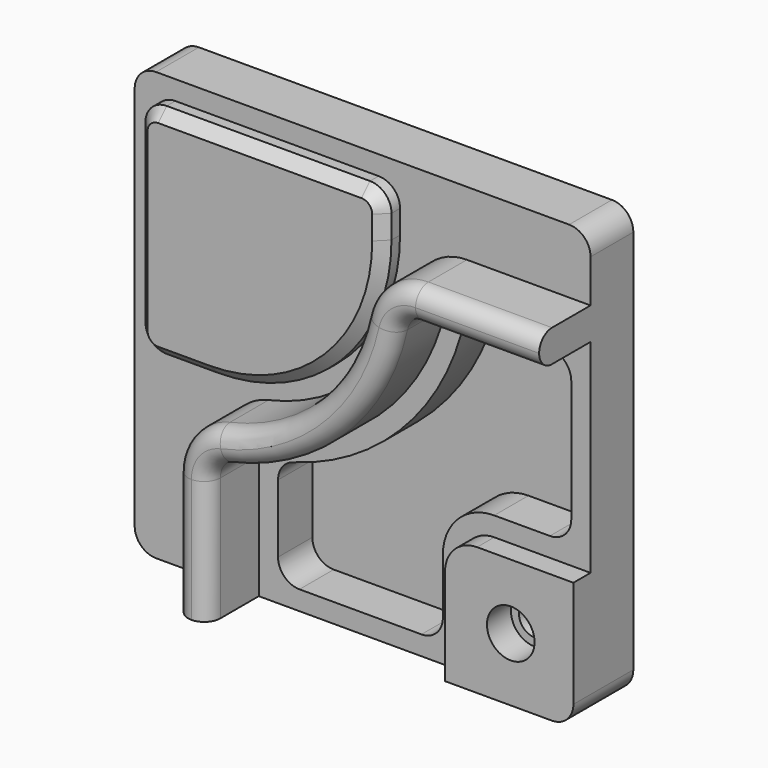
from build123d import *

# Parameters (mm, degrees)
F1_DEPTH       = 25
F2_DEPTH       = 10
F3_DEPTH       = 30
F4_DEPTH       = 20
F5_DEPTH       = 10
F7_D           = 14.75
F7_CBORE_D     = 22.25
F7_CBORE_DEPTH = 14
F8_SIZE        = 5
F9_R           = 7.49999


# Not quite as in the source:
# - a fillet or chamfer is up to 0.001 mm smaller than in the source, because OpenCascade refuses the exact size


with BuildPart() as f1:
    # F0 (on Front) → F1 (new body)
    with BuildSketch(Plane.XZ):
        with BuildLine():
            Line((96.5, 100), (-96.5, 100))
            ThreePointArc((-96.5, 100), (-103.5710678119, 97.0710678119), (-106.5, 90))
            Line((-106.5, 90), (-106.5, -90))
            ThreePointArc((-106.5, -90), (-103.5710678119, -97.0710678119), (-96.5, -100))
            Line((-96.5, -100), (-63.5, -100))
            Line((-63.5, -100), (-63.5, -42.2497216032))
            ThreePointArc((-63.5, -42.2497216032), (-58.0047374401, -26.6111405489), (-43.9347826087, -17.8476082112))
            ThreePointArc((-43.9347826087, -17.8476082112), (0.1396103068, 6.3603896932), (24.3476082112, 50.4347826087))
            ThreePointArc((24.3476082112, 50.4347826087), (33.1111405489, 64.5047374401), (48.7497216032, 70))
            Line((48.7497216032, 70), (106.5, 70))
            Line((106.5, 70), (106.5, 90))
            ThreePointArc((106.5, 90), (103.5710678119, 97.0710678119), (96.5, 100))
        make_face()
        with BuildLine():
            ThreePointArc((17.5, 70), (-6.2243507239, 12.7243507239), (-63.5, -11))
            Line((-63.5, -11), (-87.5, -11))
            ThreePointArc((-87.5, -11), (-94.5710678119, -8.0710678119), (-97.5, -1))
            Line((-97.5, -1), (-97.5, 81))
            ThreePointArc((-97.5, 81), (-94.5710678119, 88.0710678119), (-87.5, 91))
            Line((-87.5, 91), (7.5, 91))
            ThreePointArc((7.5, 91), (14.5710678119, 88.0710678119), (17.5, 81))
            Line((17.5, 81), (17.5, 70))
        make_face(mode=Mode.SUBTRACT)
        with BuildLine():
            Line((106.5, 55), (106.5, 70))
            Line((106.5, 70), (48.7497216032, 70))
            ThreePointArc((48.7497216032, 70), (33.1111405489, 64.5047374401), (24.3476082112, 50.4347826087))
            ThreePointArc((24.3476082112, 50.4347826087), (0.1396103068, 6.3603896932), (-43.9347826087, -17.8476082112))
            ThreePointArc((-43.9347826087, -17.8476082112), (-58.0047374401, -26.6111405489), (-63.5, -42.2497216032))
            Line((-63.5, -42.2497216032), (-63.5, -100))
            Line((-63.5, -100), (-48.5, -100))
            Line((-48.5, -100), (-48.5, -42.2497216032))
            ThreePointArc((-48.5, -42.2497216032), (-46.3018949761, -35.9942891815), (-40.6739130435, -32.4888762464))
            ThreePointArc((-40.6739130435, -32.4888762464), (10.7462120246, -4.2462120246), (38.9888762464, 47.1739130435))
            ThreePointArc((38.9888762464, 47.1739130435), (42.4942891815, 52.8018949761), (48.7497216032, 55))
            Line((48.7497216032, 55), (106.5, 55))
        make_face()
        with BuildLine():
            Line((106.5, -40), (106.5, 55))
            Line((106.5, 55), (48.7497216032, 55))
            ThreePointArc((48.7497216032, 55), (42.4942891815, 52.8018949761), (38.9888762464, 47.1739130435))
            ThreePointArc((38.9888762464, 47.1739130435), (10.7462120246, -4.2462120246), (-40.6739130435, -32.4888762464))
            ThreePointArc((-40.6739130435, -32.4888762464), (-46.3018949761, -35.9942891815), (-48.5, -42.2497216032))
            Line((-48.5, -42.2497216032), (-48.5, -100))
            Line((-48.5, -100), (46.5, -100))
            Line((46.5, -100), (46.5, -55))
            ThreePointArc((46.5, -55), (50.8933982822, -44.3933982822), (61.5, -40))
            Line((61.5, -40), (106.5, -40))
        make_face()
        with BuildLine():
            ThreePointArc((46.130896205, 38.7419354839), (49.7234965193, 43.981834214), (55.7476414861, 46))
            Line((55.7476414861, 46), (87.5, 46))
            ThreePointArc((87.5, 46), (94.5710678119, 43.0710678119), (97.5, 36))
            Line((97.5, 36), (97.5, -21))
            ThreePointArc((97.5, -21), (94.5710678119, -28.0710678119), (87.5, -31))
            Line((87.5, -31), (61.5, -31))
            ThreePointArc((61.5, -31), (44.5294372515, -38.0294372515), (37.5, -55))
            Line((37.5, -55), (37.5, -81))
            ThreePointArc((37.5, -81), (34.5710678119, -88.0710678119), (27.5, -91))
            Line((27.5, -91), (-29.5, -91))
            ThreePointArc((-29.5, -91), (-36.5710678119, -88.0710678119), (-39.5, -81))
            Line((-39.5, -81), (-39.5, -49.2476414861))
            ThreePointArc((-39.5, -49.2476414861), (-37.481834214, -43.2234965193), (-32.2419354839, -39.630896205))
            ThreePointArc((-32.2419354839, -39.630896205), (17.1101730553, -10.6101730553), (46.130896205, 38.7419354839))
        make_face(mode=Mode.SUBTRACT)
        with BuildLine():
            Line((106.5, -90), (106.5, -40))
            Line((106.5, -40), (61.5, -40))
            ThreePointArc((61.5, -40), (50.8933982822, -44.3933982822), (46.5, -55))
            Line((46.5, -55), (46.5, -100))
            Line((46.5, -100), (96.5, -100))
            ThreePointArc((96.5, -100), (103.5710678119, -97.0710678119), (106.5, -90))
        make_face()
        with BuildLine():
            Line((-87.5, -11), (-63.5, -11))
            ThreePointArc((-63.5, -11), (-6.2243507239, 12.7243507239), (17.5, 70))
            Line((17.5, 70), (17.5, 81))
            ThreePointArc((17.5, 81), (14.5710678119, 88.0710678119), (7.5, 91))
            Line((7.5, 91), (-87.5, 91))
            ThreePointArc((-87.5, 91), (-94.5710678119, 88.0710678119), (-97.5, 81))
            Line((-97.5, 81), (-97.5, -1))
            ThreePointArc((-97.5, -1), (-94.5710678119, -8.0710678119), (-87.5, -11))
        make_face()
        with BuildLine():
            Line((87.5, 46), (55.7476414861, 46))
            ThreePointArc((55.7476414861, 46), (49.7234965193, 43.981834214), (46.130896205, 38.7419354839))
            ThreePointArc((46.130896205, 38.7419354839), (17.1101730553, -10.6101730553), (-32.2419354839, -39.630896205))
            ThreePointArc((-32.2419354839, -39.630896205), (-37.481834214, -43.2234965193), (-39.5, -49.2476414861))
            Line((-39.5, -49.2476414861), (-39.5, -81))
            ThreePointArc((-39.5, -81), (-36.5710678119, -88.0710678119), (-29.5, -91))
            Line((-29.5, -91), (27.5, -91))
            ThreePointArc((27.5, -91), (34.5710678119, -88.0710678119), (37.5, -81))
            Line((37.5, -81), (37.5, -55))
            ThreePointArc((37.5, -55), (44.5294372515, -38.0294372515), (61.5, -31))
            Line((61.5, -31), (87.5, -31))
            ThreePointArc((87.5, -31), (94.5710678119, -28.0710678119), (97.5, -21))
            Line((97.5, -21), (97.5, 36))
            ThreePointArc((97.5, 36), (94.5710678119, 43.0710678119), (87.5, 46))
        make_face()
    extrude(amount=-F1_DEPTH)

    # F0 (on Front) → F2 (join)
    with BuildSketch(Plane.XZ):
        with BuildLine():
            Line((-87.5, -11), (-63.5, -11))
            ThreePointArc((-63.5, -11), (-6.2243507239, 12.7243507239), (17.5, 70))
            Line((17.5, 70), (17.5, 81))
            ThreePointArc((17.5, 81), (14.5710678119, 88.0710678119), (7.5, 91))
            Line((7.5, 91), (-87.5, 91))
            ThreePointArc((-87.5, 91), (-94.5710678119, 88.0710678119), (-97.5, 81))
            Line((-97.5, 81), (-97.5, -1))
            ThreePointArc((-97.5, -1), (-94.5710678119, -8.0710678119), (-87.5, -11))
        make_face()
    extrude(amount=F2_DEPTH)

    # F0 (on Front) → F3 (join)
    with BuildSketch(Plane.XZ):
        with BuildLine():
            Line((106.5, 55), (106.5, 70))
            Line((106.5, 70), (48.7497216032, 70))
            ThreePointArc((48.7497216032, 70), (33.1111405489, 64.5047374401), (24.3476082112, 50.4347826087))
            ThreePointArc((24.3476082112, 50.4347826087), (0.1396103068, 6.3603896932), (-43.9347826087, -17.8476082112))
            ThreePointArc((-43.9347826087, -17.8476082112), (-58.0047374401, -26.6111405489), (-63.5, -42.2497216032))
            Line((-63.5, -42.2497216032), (-63.5, -100))
            Line((-63.5, -100), (-48.5, -100))
            Line((-48.5, -100), (-48.5, -42.2497216032))
            ThreePointArc((-48.5, -42.2497216032), (-46.3018949761, -35.9942891815), (-40.6739130435, -32.4888762464))
            ThreePointArc((-40.6739130435, -32.4888762464), (10.7462120246, -4.2462120246), (38.9888762464, 47.1739130435))
            ThreePointArc((38.9888762464, 47.1739130435), (42.4942891815, 52.8018949761), (48.7497216032, 55))
            Line((48.7497216032, 55), (106.5, 55))
        make_face()
    extrude(amount=F3_DEPTH)

    # F0 (on Front) → F4 (cut)
    with BuildSketch(Plane.XZ):
        with BuildLine():
            Line((87.5, 46), (55.7476414861, 46))
            ThreePointArc((55.7476414861, 46), (49.7234965193, 43.981834214), (46.130896205, 38.7419354839))
            ThreePointArc((46.130896205, 38.7419354839), (17.1101730553, -10.6101730553), (-32.2419354839, -39.630896205))
            ThreePointArc((-32.2419354839, -39.630896205), (-37.481834214, -43.2234965193), (-39.5, -49.2476414861))
            Line((-39.5, -49.2476414861), (-39.5, -81))
            ThreePointArc((-39.5, -81), (-36.5710678119, -88.0710678119), (-29.5, -91))
            Line((-29.5, -91), (27.5, -91))
            ThreePointArc((27.5, -91), (34.5710678119, -88.0710678119), (37.5, -81))
            Line((37.5, -81), (37.5, -55))
            ThreePointArc((37.5, -55), (44.5294372515, -38.0294372515), (61.5, -31))
            Line((61.5, -31), (87.5, -31))
            ThreePointArc((87.5, -31), (94.5710678119, -28.0710678119), (97.5, -21))
            Line((97.5, -21), (97.5, 36))
            ThreePointArc((97.5, 36), (94.5710678119, 43.0710678119), (87.5, 46))
        make_face()
    extrude(amount=-F4_DEPTH, mode=Mode.SUBTRACT)

    # F0 (on Front) → F5 (join)
    with BuildSketch(Plane.XZ):
        with BuildLine():
            Line((106.5, -90), (106.5, -40))
            Line((106.5, -40), (61.5, -40))
            ThreePointArc((61.5, -40), (50.8933982822, -44.3933982822), (46.5, -55))
            Line((46.5, -55), (46.5, -100))
            Line((46.5, -100), (96.5, -100))
            ThreePointArc((96.5, -100), (103.5710678119, -97.0710678119), (106.5, -90))
        make_face()
    extrude(amount=F5_DEPTH)

    # F7 (through all)
    with Locations(Plane.XZ.offset(10)):
        with Locations((77.2273465991, -70.3643187881)):
            CounterBoreHole(F7_D / 2, F7_CBORE_D / 2, F7_CBORE_DEPTH)

    # F8
    f8_edges = [f1.edges().sort_by_distance(p)[0] for p in [
        (-97.5, -10, 40),
    ]]
    chamfer(f8_edges, length=F8_SIZE)

    # F9 (radius 7.5 in the source; OpenCascade refuses exactly that, so slightly less here)
    f9_edges = [f1.edges().sort_by_distance(p)[0] for p in [
        (-63.5, -30, -71.124861),
        (-48.5, -30, -71.124861),
    ]]
    fillet(f9_edges, radius=F9_R)


solid = f1.part
